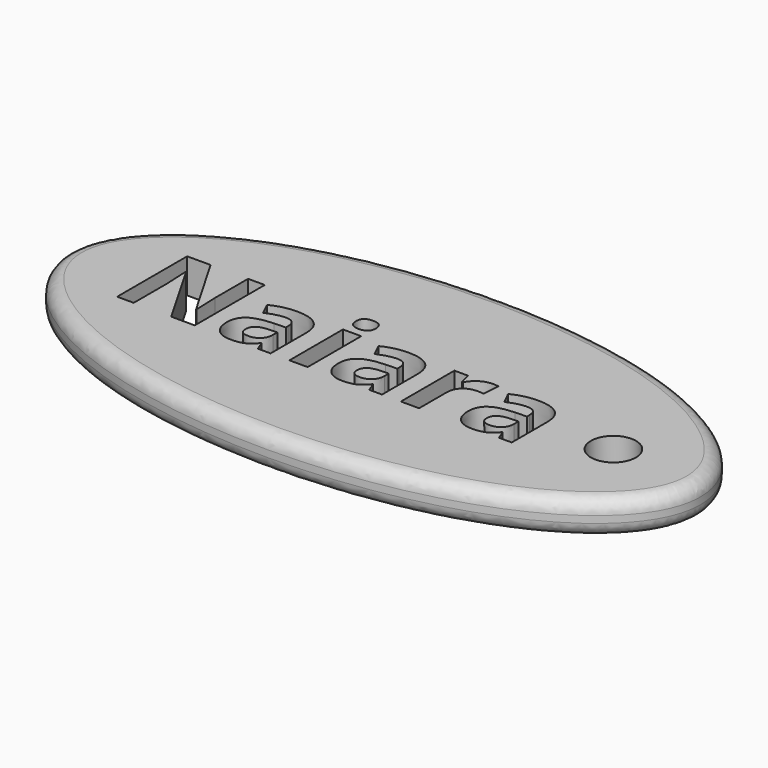
from build123d import *

# Parameters (mm, degrees)
F1_DEPTH     = 3.81
F2_R         = 1.524
F3_R         = 2.4917157379
F3_TEXT_SIZE = 13.5510582133
F4_DEPTH     = 3.8110001


# Not quite as in the source:
# - Text() gives the source's letters only with a copy of the font that has no kerning and outlines rounded to 1/6400 em; it was checked with that copy


with BuildPart() as f1:
    # F0 (on Top) → F1 (new body)
    with BuildSketch(Plane.XY):
        with BuildLine():
            add(Edge.make_bspline(
                [(34.9683985114, 0), (34.9683985114, 28.4775254861), (-17.4841992557, 14.238762743), (-69.9367970228, 0), (-17.4841992557, -14.238762743), (34.9683985114, -28.4775254861), (34.9683985114, 0)],
                knots=[0, 0, 0, 2.0943951024, 2.0943951024, 4.1887902048, 4.1887902048, 6.2831853072, 6.2831853072, 6.2831853072], degree=2, weights=[1, 0.5, 1, 0.5, 1, 0.5, 1]))
        make_face()
    extrude(amount=F1_DEPTH)

    # F2
    f2_edges = [f1.edges().sort_by_distance(p)[0] for p in [
        (-34.968399, 9e-06, 3.81),
        (-34.968399, 9e-06, 0),
    ]]
    fillet(f2_edges, radius=F2_R)

    # F3 (on face) → F4 (cut, through all)
    with BuildSketch(Plane.XY.offset(3.81)):
        with Locations((25.3600347787, 0)):
            Circle(F3_R)
        with Locations((-27.1174784471, -4.5055614524)):
            Text('Naiara', F3_TEXT_SIZE, font='Open Sans', font_style=FontStyle.BOLD, text_align=(TextAlign.LEFT, TextAlign.BOTTOM))
    extrude(amount=-F4_DEPTH, mode=Mode.SUBTRACT)


solid = f1.part
